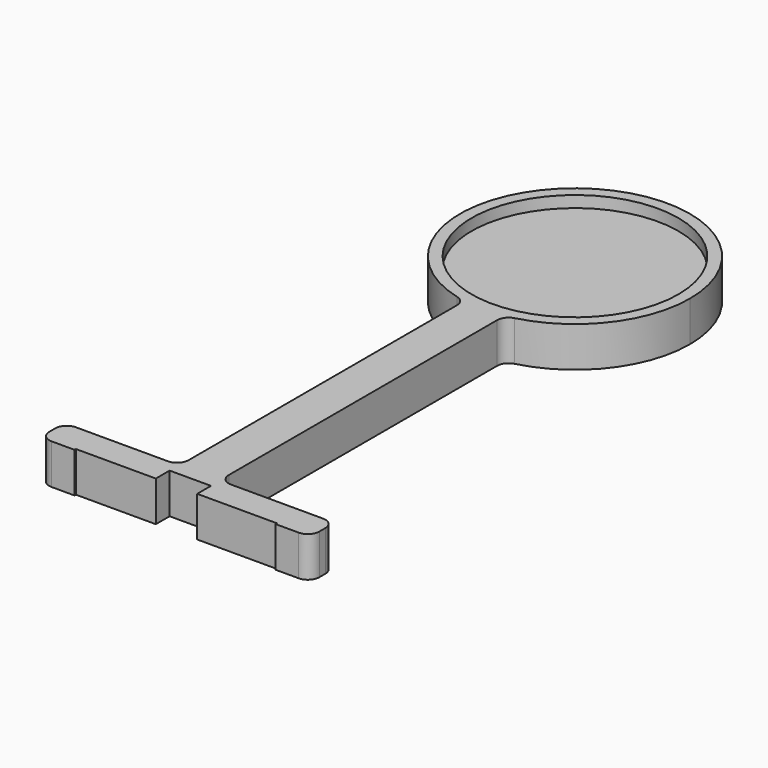
from build123d import *

# Parameters (mm, degrees)
F0_W     = 6
F0_H     = 0.3
F1_DEPTH = 7
F2_R     = 18
F3_DEPTH = 2
F4_R     = 2


# Not quite as in the source:
# - a feature names something its author has since deleted; it is built from what else it names


with BuildPart() as f1:
    # F0 (on Top) → F1 (new body)
    with BuildSketch(Plane.XY):
        with BuildLine():
            ThreePointArc((3.5, -3), (0, -3.3086313325), (-3.5, -3))
            Line((-3.5, -3), (-3.5, -65))
            Line((-3.5, -65), (-23.5, -65))
            Line((-23.5, -65), (-23.5, -70))
            Line((-23.5, -70), (-17.5, -70))
            Line((-17.5, -70), (-3.6, -70))
            Line((-3.6, -70), (-3.6, -67))
            Line((-3.6, -67), (3.6, -67))
            Line((3.6, -67), (3.6, -70))
            Line((3.6, -70), (17.5, -70))
            Line((17.5, -70), (23.5, -70))
            Line((23.5, -70), (23.5, -65))
            Line((23.5, -65), (3.5, -65))
            Line((3.5, -65), (3.5, -3))
        make_face()
        with BuildLine():
            ThreePointArc((20, 16.6913686675), (-12.8452325787, 32.0210783843), (-3.5, -3))
            ThreePointArc((-3.5, -3), (0, -3.3086313325), (3.5, -3))
            ThreePointArc((3.5, -3), (15.3297097168, 3.8461360889), (20, 16.6913686675))
        make_face()
        with Locations((-20.5, -70.15)):
            Rectangle(F0_W, F0_H)
        with Locations((20.5, -70.15)):
            Rectangle(F0_W, F0_H)
    extrude(amount=F1_DEPTH)

    # F2 (on face) → F3 (cut)
    with BuildSketch(Plane.XY.offset(7)):
        with Locations((0, 16.6913686675)):
            Circle(F2_R)
    extrude(amount=-F3_DEPTH, mode=Mode.SUBTRACT)

    # F4
    f4_edges = [f1.edges().sort_by_distance(p)[0] for p in [
        (-3.5, -3, 3.5),
        (3.5, -3, 3.5),
        (23.5, -65, 3.5),
        (-23.5, -65, 3.5),
        (-3.5, -65, 3.5),
        (3.5, -65, 3.5),
        (-23.5, -70.3, 3.5),
        (23.5, -70.3, 3.5),
    ]]
    fillet(f4_edges, radius=F4_R)


solid = f1.part
